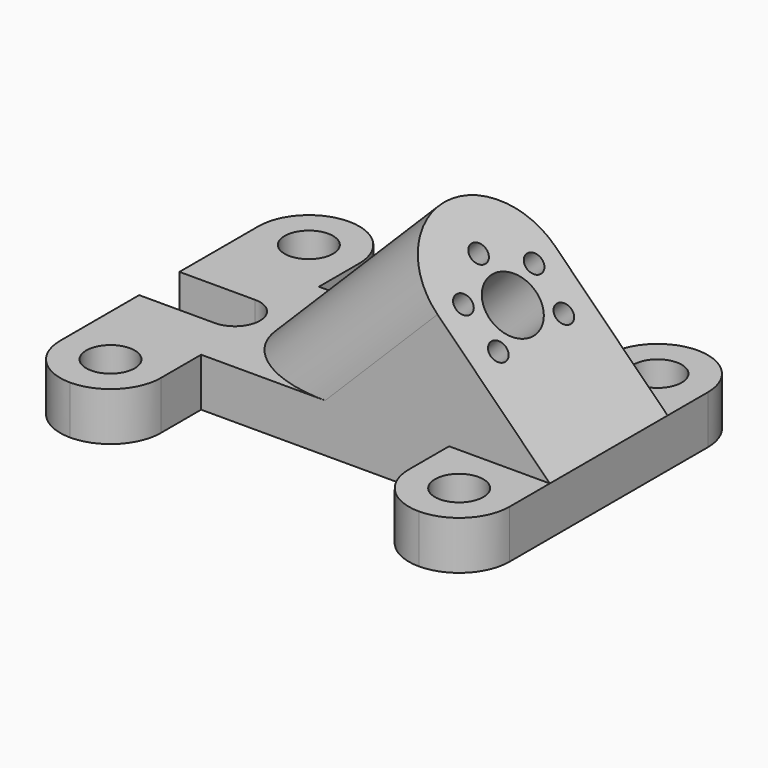
from build123d import *

# Parameters (mm, degrees)
F1_DEPTH  = 90
F2_W      = 64
F2_H      = 26
F3_DEPTH  = 100
F4_W      = 26
F4_H      = 26
F5_DEPTH  = 100
F6_W      = 26
F6_H      = 26
F7_DEPTH  = 105
F8_R      = 12.99999
F9_R      = 18.99999
F10_R     = 7.5
F10_R_2   = 2.5
F11_DEPTH = 25
F13_DEPTH = 25
F15_DEPTH = 25
F17_DEPTH = 25
F19_DEPTH = 25
F20_R     = 7.5
F21_DEPTH = 100


# Not quite as in the source:
# - a fillet or chamfer is up to 0.001 mm smaller than in the source, because OpenCascade refuses the exact size


with BuildPart() as f1:
    # F0 (on Front) → F1 (new body)
    with BuildSketch(Plane.XZ):
        Polygon((0, 12.5), (0, 0), (116, 0), (116, 12.5), (73.5735931288, 54.9264068712), (31.1471862576, 12.5), align=None)
    extrude(amount=F1_DEPTH)

    # F2 (on face) → F3 (cut)
    with BuildSketch(Plane(origin=(0, 0, 0), x_dir=(1, 0, 0), z_dir=(0, 0, -1))):
        with Locations((58, 77)):
            Rectangle(F2_W, F2_H)
        with Locations((58, 13)):
            Rectangle(F2_W, F2_H)
    extrude(amount=-F3_DEPTH, mode=Mode.SUBTRACT)

    # F4 (on face) → F5 (cut)
    with BuildSketch(Plane(origin=(90, 0, 0), x_dir=(0, -1, 0), z_dir=(-1, 0, 0))):
        with Locations((13, 25.5)):
            Rectangle(F4_W, F4_H)
    extrude(amount=-F5_DEPTH, mode=Mode.SUBTRACT)

    # F6 (on face) → F7 (cut)
    with BuildSketch(Plane(origin=(90, 0, 0), x_dir=(0, -1, 0), z_dir=(-1, 0, 0))):
        with Locations((77, 25.5)):
            Rectangle(F6_W, F6_H)
    extrude(amount=-F7_DEPTH, mode=Mode.SUBTRACT)

    # F8 (radius 13 in the source; OpenCascade refuses exactly that, so slightly less here)
    f8_edges = [f1.edges().sort_by_distance(p)[0] for p in [
        (0, 0, 6.25),
        (26, 0, 6.25),
        (116, -90, 6.25),
        (90, -90, 6.25),
        (26, -90, 6.25),
        (0, -90, 6.25),
        (116, 0, 6.25),
        (90, 0, 6.25),
    ]]
    fillet(f8_edges, radius=F8_R)

    # F9 (radius 19 in the source; OpenCascade refuses exactly that, so slightly less here)
    f9_edges = [f1.edges().sort_by_distance(p)[0] for p in [
        (52.36039, -64, 33.713203),
        (52.36039, -26, 33.713203),
    ]]
    fillet(f9_edges, radius=F9_R)

    # F10 (on face) → F11 (cut)
    with BuildSketch(Plane(origin=(64.25, 0, 64.25), x_dir=(0, 1, 0), z_dir=(0.7071067812, 0, 0.7071067812))):
        with Locations((-45, -38.1855518528)):
            Circle(F10_R)
        with Locations((-45, -25.6855518528)):
            Circle(F10_R_2)
        with Locations((-33.6018534744, -33.0540554063)):
            Circle(F10_R_2)
        with Locations((-56.3981465256, -33.0540554063)):
            Circle(F10_R_2)
        with Locations((-55.573814617, -44.8522185195)):
            Circle(F10_R_2)
        with Locations((-34.426185383, -44.8522185195)):
            Circle(F10_R_2)
    extrude(amount=-F11_DEPTH, mode=Mode.SUBTRACT)

    # F12 (on face) → F13 (cut)
    with BuildSketch(Plane.XY.offset(12.5)):
        with BuildLine():
            ThreePointArc((6.75, -13), (13, -19.25), (19.25, -13))
            ThreePointArc((19.25, -13), (13, -6.75), (6.75, -13))
        make_face()
        with BuildLine():
            ThreePointArc((6.75, -77), (13, -83.25), (19.25, -77))
            ThreePointArc((19.25, -77), (13, -70.75), (6.75, -77))
        make_face()
    extrude(amount=-F13_DEPTH, mode=Mode.SUBTRACT)

    # F14 (on face) → F15 (cut)
    with BuildSketch(Plane.XY.offset(12.5)):
        with BuildLine():
            ThreePointArc((96.75, -13), (103, -19.25), (109.25, -13))
            ThreePointArc((109.25, -13), (103, -6.75), (96.75, -13))
        make_face()
    extrude(amount=-F15_DEPTH, mode=Mode.SUBTRACT)

    # F16 (on face) → F17 (cut)
    with BuildSketch(Plane.XY.offset(12.5)):
        with BuildLine():
            ThreePointArc((96.75, -77), (103, -83.25), (109.25, -77))
            ThreePointArc((109.25, -77), (103, -70.75), (96.75, -77))
        make_face()
    extrude(amount=-F17_DEPTH, mode=Mode.SUBTRACT)

    # F18 (on face) → F19 (cut)
    with BuildSketch(Plane.XY.offset(12.5)):
        with BuildLine():
            Line((19.5, -38.5), (0, -38.5))
            Line((0, -38.5), (0, -45))
            Line((0, -45), (0, -51.5))
            Line((0, -51.5), (19.5, -51.5))
            ThreePointArc((19.5, -51.5), (24.0961940777, -49.5961940777), (26, -45))
            ThreePointArc((26, -45), (24.0961940777, -40.4038059223), (19.5, -38.5))
        make_face()
    extrude(amount=-F19_DEPTH, mode=Mode.SUBTRACT)

    # F20 (on face) → F21 (cut)
    with BuildSketch(Plane(origin=(64.25, 0, 64.25), x_dir=(0, 1, 0), z_dir=(0.7071067812, 0, 0.7071067812))):
        with Locations((-45, -38.1855518528)):
            Circle(F20_R)
    extrude(amount=-F21_DEPTH, mode=Mode.SUBTRACT)


solid = f1.part
